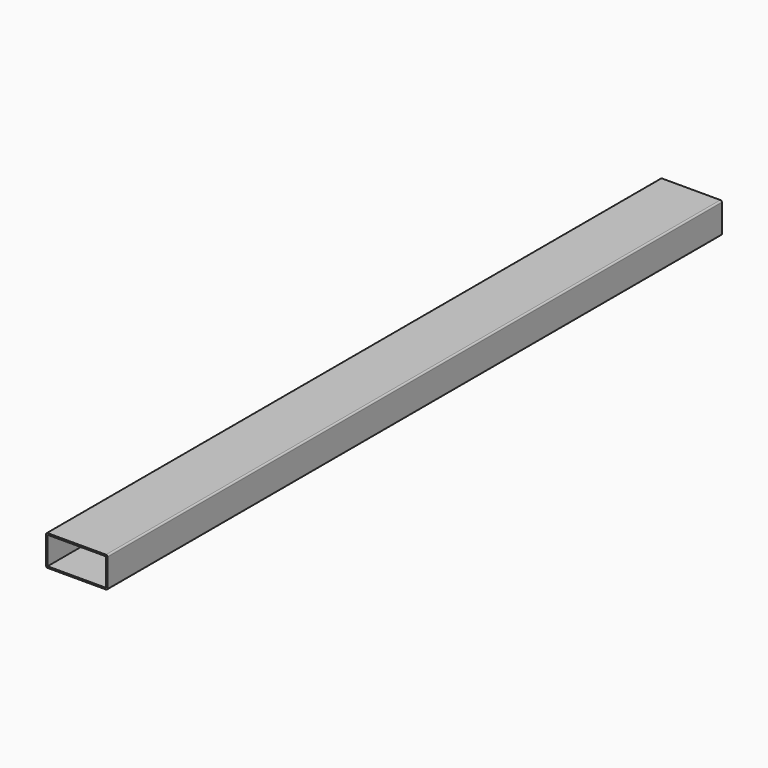
from build123d import *

# Parameters (mm, degrees)
F0_W     = 76
F0_H     = 36
F1_DEPTH = 1000


# Not quite as in the source:
# - ends of sketch curves that miss each other by under 0.0002 mm in the source are joined


with BuildPart() as f1:
    # F0 (on Front) → F1 (new body)
    with BuildSketch(Plane.XZ):
        with BuildLine():
            ThreePointArc((-37.999999, 20), (-39.4142135624, 19.4142135624), (-40, 17.999999))
            Line((-40, 17.999999), (-40, -18))
            ThreePointArc((-40, -18), (-39.4142128553, -19.4142142695), (-37.999999, -20))
            Line((-37.999999, -20), (38, -20))
            ThreePointArc((38, -20), (39.4142139159, -19.4142132088), (40, -18))
            Line((40, -18), (40, 18))
            ThreePointArc((40, 18), (39.4142139159, 19.4142132088), (38.000001, 20))
            Line((38.000001, 20), (-37.999999, 20))
        make_face()
        Rectangle(F0_W, F0_H, mode=Mode.SUBTRACT)
    extrude(amount=F1_DEPTH)


solid = f1.part
